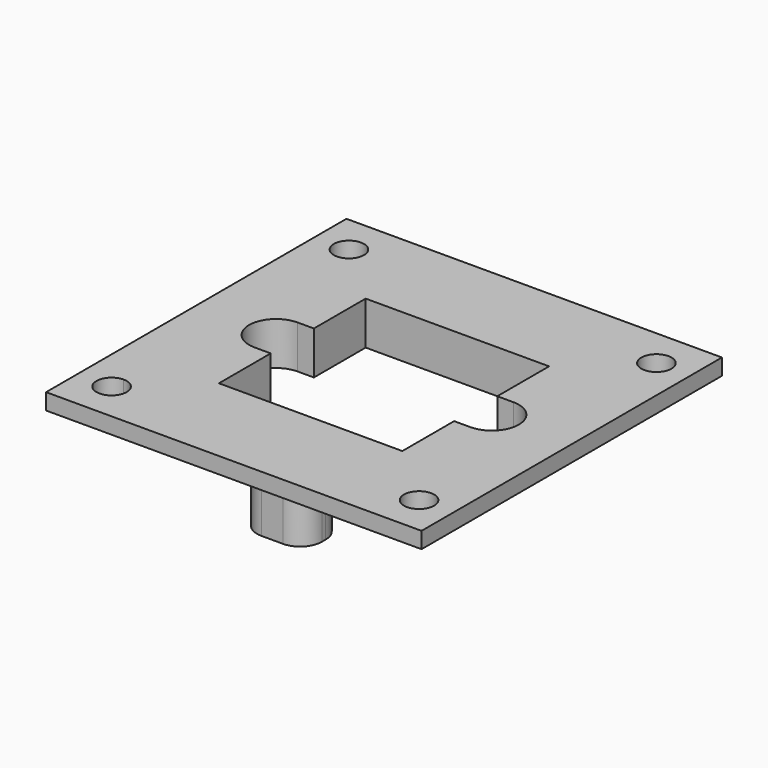
from build123d import *

# Parameters (mm, degrees)
F0_R     = 13.3
F1_DEPTH = 4
F2_W     = 6
F2_H     = 4.4572373599
F3_DEPTH = 4.2
F4_R     = 2
F5_R     = 1.4
F6_DEPTH = 1.5


with BuildPart() as f1:
    # F0 (on Top) → F1 (new body)
    with BuildSketch(Plane.XY):
        Circle(F0_R)
        with BuildLine():
            Line((0, -8.5), (-8.5, -8.5))
            Line((-8.5, -8.5), (-8.5, -2.5))
            Line((-8.5, -2.5), (-10, -2.5))
            ThreePointArc((-10, -2.5), (-12.5, 0), (-10, 2.5))
            Line((-10, 2.5), (-8.5, 2.5))
            Line((-8.5, 2.5), (-8.5, 8.5))
            Line((-8.5, 8.5), (0, 8.5))
            Line((0, 8.5), (8.5, 8.5))
            Line((8.5, 8.5), (8.5, 2.5))
            Line((8.5, 2.5), (10, 2.5))
            ThreePointArc((10, 2.5), (11.767766953, 1.767766953), (12.5, 0))
            ThreePointArc((12.5, 0), (11.767766953, -1.767766953), (10, -2.5))
            Line((10, -2.5), (8.5, -2.5))
            Line((8.5, -2.5), (8.5, -8.5))
            Line((8.5, -8.5), (0, -8.5))
        make_face(mode=Mode.SUBTRACT)
    extrude(amount=F1_DEPTH)

    # F2 (on face) → F3 (join)
    with BuildSketch(Plane(origin=(0, 0, 0), x_dir=(1, 0, 0), z_dir=(0, 0, -1))):
        with Locations((0, 10.7286186799)):
            Rectangle(F2_W, F2_H)
    extrude(amount=F3_DEPTH)

    # F4
    f4_edges = [f1.edges().sort_by_distance(p)[0] for p in [
        (-3, -12.957237, -2.1),
        (-3, -8.5, -2.1),
        (3, -8.5, -2.1),
        (3, -12.957237, -2.1),
    ]]
    fillet(f4_edges, radius=F4_R)

    # F5 (on face) → F6 (join)
    with BuildSketch(Plane.XY.offset(4)):
        with BuildLine():
            ThreePointArc((0, 13.3), (9.4045201898, 9.4045201898), (13.3, 0))
            ThreePointArc((13.3, 0), (9.4045201898, -9.4045201898), (0, -13.3))
            Line((0, -13.3), (0, -13.75))
            Line((0, -13.75), (0, -17.4))
            Line((0, -17.4), (17.4, -17.4))
            Line((17.4, -17.4), (17.4, 17.4))
            Line((17.4, 17.4), (0, 17.4))
            Line((0, 17.4), (0, 13.3))
        make_face()
        with BuildLine():
            ThreePointArc((15.65, -13.75), (14.25, -15.15), (12.85, -13.75))
            ThreePointArc((12.85, -13.75), (14.25, -12.35), (15.65, -13.75))
        make_face(mode=Mode.SUBTRACT)
        with Locations((14.25, 13.75)):
            Circle(F5_R, mode=Mode.SUBTRACT)
        with BuildLine():
            Line((0, 8.5), (0, 13.3))
            ThreePointArc((0, 13.3), (-9.4045201898, 9.4045201898), (-13.3, 0))
            Line((-13.3, 0), (-12.5, 0))
            ThreePointArc((-12.5, 0), (-11.767766953, 1.767766953), (-10, 2.5))
            Line((-10, 2.5), (-8.5, 2.5))
            Line((-8.5, 2.5), (-8.5, 8.5))
            Line((-8.5, 8.5), (0, 8.5))
        make_face()
        with BuildLine():
            ThreePointArc((-13.3, 0), (-9.4045201898, 9.4045201898), (0, 13.3))
            Line((0, 13.3), (0, 17.4))
            Line((0, 17.4), (-17.4, 17.4))
            Line((-17.4, 17.4), (-17.4, -17.4))
            Line((-17.4, -17.4), (0, -17.4))
            Line((0, -17.4), (0, -13.75))
            Line((0, -13.75), (-12.85, -13.75))
            ThreePointArc((-12.85, -13.75), (-15.2399494937, -14.7399494937), (-14.25, -12.35))
            Line((-14.25, -12.35), (-14.25, 0))
            Line((-14.25, 0), (-13.3, 0))
        make_face()
        with BuildLine():
            ThreePointArc((-12.85, 13.75), (-13.2600505063, 12.7600505063), (-14.25, 12.35))
            ThreePointArc((-14.25, 12.35), (-15.2399494937, 14.7399494937), (-12.85, 13.75))
        make_face(mode=Mode.SUBTRACT)
        with BuildLine():
            Line((0, -13.75), (0, -13.3))
            ThreePointArc((0, -13.3), (-9.4045201898, -9.4045201898), (-13.3, 0))
            Line((-13.3, 0), (-14.25, 0))
            Line((-14.25, 0), (-14.25, -12.35))
            ThreePointArc((-14.25, -12.35), (-13.2600505063, -12.7600505063), (-12.85, -13.75))
            Line((-12.85, -13.75), (0, -13.75))
        make_face()
        with BuildLine():
            ThreePointArc((-13.3, 0), (-9.4045201898, -9.4045201898), (0, -13.3))
            Line((0, -13.3), (0, -8.5))
            Line((0, -8.5), (-8.5, -8.5))
            Line((-8.5, -8.5), (-8.5, -2.5))
            Line((-8.5, -2.5), (-10, -2.5))
            ThreePointArc((-10, -2.5), (-11.767766953, -1.767766953), (-12.5, 0))
            Line((-12.5, 0), (-13.3, 0))
        make_face()
    extrude(amount=-F6_DEPTH)


solid = f1.part
